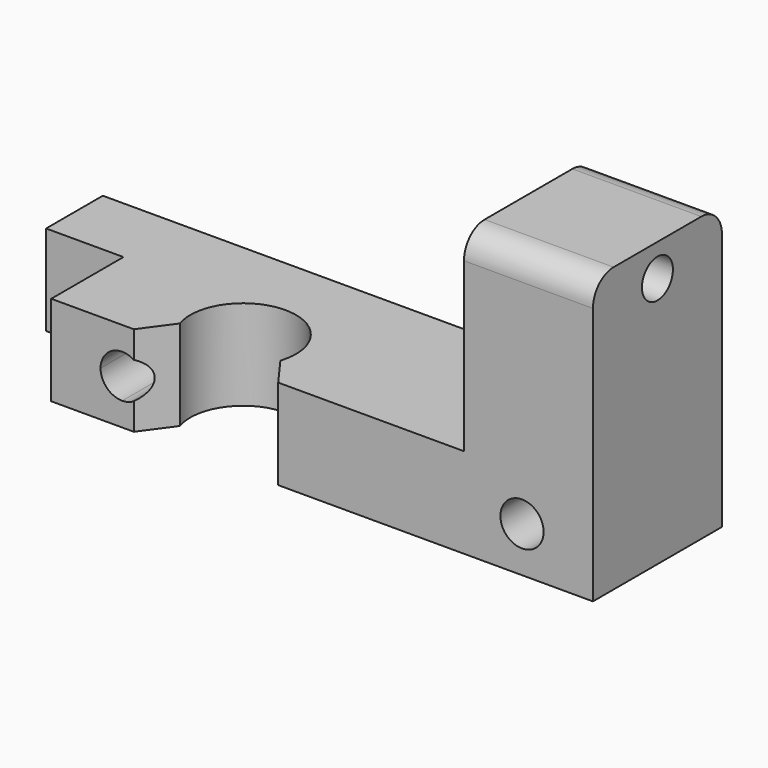
from build123d import *

# Parameters (mm, degrees)
F1_W         = 42
F1_H         = 12.5
F2_DEPTH     = 7
F3_R         = 4.1
F4_DEPTH     = 25
F5_T1_DEPTH  = 26.0282480506
F7_DEPTH     = 25
F8_TEXT_SIZE = 9.7222222222
F9_DEPTH     = 1
F10_W        = 10
F10_H        = 12.5
F11_DEPTH    = 15
F12_R        = 1.5
F13_DEPTH    = 25
F14_R        = 2
F15_W        = 5.5
F15_H        = 7
F16_DEPTH    = 6


# Not quite as in the source:
# - a fillet or chamfer that OpenCascade refuses, or shapes differently, is made with other operations: its cross-section is extruded or revolved along the edge and cut away or added
# - Text() gives the source's letters only with a copy of the font that has no kerning and outlines rounded to 1/6400 em; it was checked with that copy


with BuildPart() as f2:
    # F1 (on Top) → F2 (new body)
    with BuildSketch(Plane.XY):
        with Locations((21, 6.25)):
            Rectangle(F1_W, F1_H)
    extrude(amount=F2_DEPTH)

    # F3 (on face) → F4 (cut)
    with BuildSketch(Plane.XY.offset(7)):
        with Locations((12, 3.6)):
            Circle(F3_R)
    extrude(amount=-F4_DEPTH, mode=Mode.SUBTRACT)

    # F5: chamfer of 7 on 2 edges, made by hand

    # F5_s2 → F5_t1 (cut)
    with BuildSketch(Plane.XY.offset(-9.5141240253)):
        with BuildLine():
            Line((17.7610452751, -0.2264961011), (15.73515334, 2.5608842714))
            Line((15.73515334, 2.5608842714), (15.6019903715, 2.6041002851))
            ThreePointArc((15.6019903715, 2.6041002851), (15.0707550937, 1.0995874031), (13.895141727, 0.1229268293))
            Line((13.895141727, 0.1229268293), (13.962141687, -0.14))
            ThreePointArc((13.962141687, -0.14), (15.861593481, -0.14), (17.7610452751, -0.3664961011))
            Line((17.7610452751, -0.3664961011), (17.7610452751, -0.2264961011))
        make_face()
        with BuildLine():
            Line((8.26484666, 2.5608842714), (6.2389547249, -0.2264961011))
            Line((6.2389547249, -0.2264961011), (6.2389547249, -0.3664961011))
            ThreePointArc((6.2389547249, -0.3664961011), (8.138406519, -0.14), (10.037858313, -0.14))
            Line((10.037858313, -0.14), (10.104858273, 0.1229268293))
            ThreePointArc((10.104858273, 0.1229268293), (8.9292449063, 1.0995874031), (8.3980096285, 2.6041002851))
            Line((8.3980096285, 2.6041002851), (8.26484666, 2.5608842714))
        make_face()
    extrude(amount=F5_T1_DEPTH, mode=Mode.SUBTRACT)

    # F6 (on face) → F7 (cut)
    with BuildSketch(Plane(origin=(0, 12.5, 0), x_dir=(-1, 0, 0), z_dir=(0, 1, 0))):
        with BuildLine():
            Line((-5.5, 3.5), (-3.825, 3.5))
            ThreePointArc((-3.825, 3.5), (-4.3155961415, 4.6844038585), (-5.5, 5.175))
            Line((-5.5, 5.175), (-5.5, 3.5))
        make_face()
        with BuildLine():
            ThreePointArc((-5.5, 1.825), (-4.3155961415, 2.3155961415), (-3.825, 3.5))
            Line((-3.825, 3.5), (-5.5, 3.5))
            Line((-5.5, 3.5), (-5.5, 1.825))
        make_face()
        with BuildLine():
            Line((-5.5, 3.5), (-5.5, 5.175))
            ThreePointArc((-5.5, 5.175), (-7.175, 3.5), (-5.5, 1.825))
            Line((-5.5, 1.825), (-5.5, 3.5))
        make_face()
        with BuildLine():
            ThreePointArc((-38.175, 3.5), (-36.5, 1.825), (-34.825, 3.5))
            ThreePointArc((-34.825, 3.5), (-36.5, 5.175), (-38.175, 3.5))
        make_face()
    extrude(amount=-F7_DEPTH, mode=Mode.SUBTRACT)

    # F8 (on face) → F9 (join)
    with BuildSketch(Plane(origin=(0, 12.5, 0), x_dir=(-1, 0, 0), z_dir=(0, 1, 0))):
        with Locations((-26.2691155076, 0)):
            Text('R', F8_TEXT_SIZE, font='Open Sans', font_style=FontStyle.BOLD, text_align=(TextAlign.LEFT, TextAlign.BOTTOM))
    extrude(amount=F9_DEPTH)

    # F10 (on face) → F11 (join)
    with BuildSketch(Plane.XY.offset(7)):
        with Locations((37, 6.25)):
            Rectangle(F10_W, F10_H)
    extrude(amount=F11_DEPTH)

    # F12 (on face) → F13 (cut)
    with BuildSketch(Plane.YZ.offset(42)):
        with Locations((6.25, 19.5)):
            Circle(F12_R)
    extrude(amount=-F13_DEPTH, mode=Mode.SUBTRACT)

    # F14
    f14_edges = [f2.edges().sort_by_distance(p)[0] for p in [
        (37, 0, 22),
        (37, 12.5, 22),
    ]]
    fillet(f14_edges, radius=F14_R)

    # F15 (on face) → F16 (join)
    with BuildSketch(Plane(origin=(0, 0, 0), x_dir=(0, -1, 0), z_dir=(-1, 0, 0))):
        with Locations((-9.75, 3.5)):
            Rectangle(F15_W, F15_H)
    extrude(amount=F16_DEPTH)


solid = f2.part
